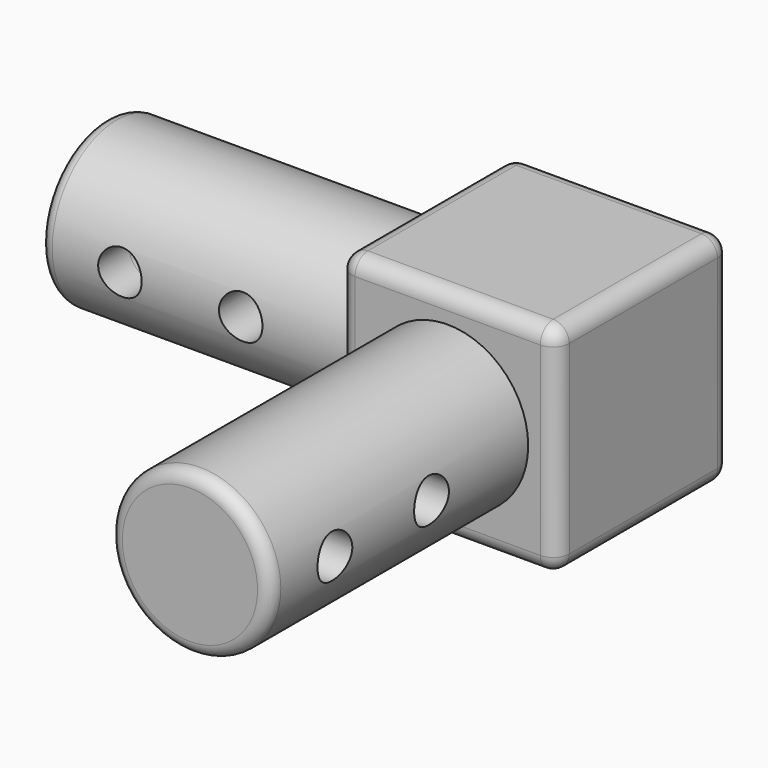
from build123d import *

# Parameters (mm, degrees)
F0_W      = 34.29
F0_H      = 34.29
F1_DEPTH  = 34.29
F2_R      = 12.7
F3_DEPTH  = 50.8
F4_R      = 12.7
F5_DEPTH  = 50.8
F6_R      = 3.429
F7_DEPTH  = 25.4
F8_R      = 3.429
F9_DEPTH  = 25.4
F10_R     = 3.429
F11_DEPTH = 25.4
F12_R     = 2.032
F13_R     = 2.54


with BuildPart() as f1:
    # F0 (on Top) → F1 (new body)
    with BuildSketch(Plane.XY):
        with Locations((3.6728888822, 6.5610635031)):
            Rectangle(F0_W, F0_H)
    extrude(amount=F1_DEPTH)

    # F2 (on face) → F3 (join)
    with BuildSketch(Plane(origin=(-13.4721111178, 0, 0), x_dir=(0, -1, 0), z_dir=(-1, 0, 0))):
        with Locations((-6.5610635031, 17.145)):
            Circle(F2_R)
    extrude(amount=F3_DEPTH)

    # F4 (on face) → F5 (join)
    with BuildSketch(Plane.XZ.offset(10.5839364969)):
        with Locations((3.6728888822, 17.145)):
            Circle(F4_R)
    extrude(amount=F5_DEPTH)

    # F6 (on Front) → F7 (cut, symmetric)
    with BuildSketch(Plane.XZ):
        with Locations((3.6728888822, 53.34)):
            Circle(F6_R)
        with Locations((3.6728888822, 72.39)):
            Circle(F6_R)
    extrude(amount=F7_DEPTH, both=True, mode=Mode.SUBTRACT)

    # F8 (on Right) → F9 (cut, symmetric)
    with BuildSketch(Plane.YZ):
        with Locations((-29.6339364969, 17.145)):
            Circle(F8_R)
        with Locations((-48.6839364969, 17.145)):
            Circle(F8_R)
    extrude(amount=F9_DEPTH, both=True, mode=Mode.SUBTRACT)

    # F10 (on Front) → F11 (cut, symmetric)
    with BuildSketch(Plane.XZ):
        with Locations((-51.5721111178, 17.145)):
            Circle(F10_R)
        with Locations((-32.5221111178, 17.145)):
            Circle(F10_R)
    extrude(amount=F11_DEPTH, both=True, mode=Mode.SUBTRACT)

    # F12
    f12_edges = [f1.edges().sort_by_distance(p)[0] for p in [
        (-9.027111, -61.383936, 17.145),
        (-64.272111, 19.261064, 17.145),
    ]]
    fillet(f12_edges, radius=F12_R)

    # F13
    f13_edges = [f1.edges().sort_by_distance(p)[0] for p in [
        (20.817889, 23.706064, 17.145),
        (20.817889, 6.561064, 34.29),
        (20.817889, -10.583936, 17.145),
        (20.817889, 6.561064, 0),
        (3.672889, 23.706064, 0),
        (3.672889, 23.706064, 34.29),
        (-13.472111, 23.706064, 17.145),
        (-13.472111, 6.561064, 0),
        (3.672889, -10.583936, 0),
        (-13.472111, 6.561064, 34.29),
        (-13.472111, -10.583936, 17.145),
        (3.672889, -10.583936, 34.29),
    ]]
    fillet(f13_edges, radius=F13_R)


solid = f1.part
